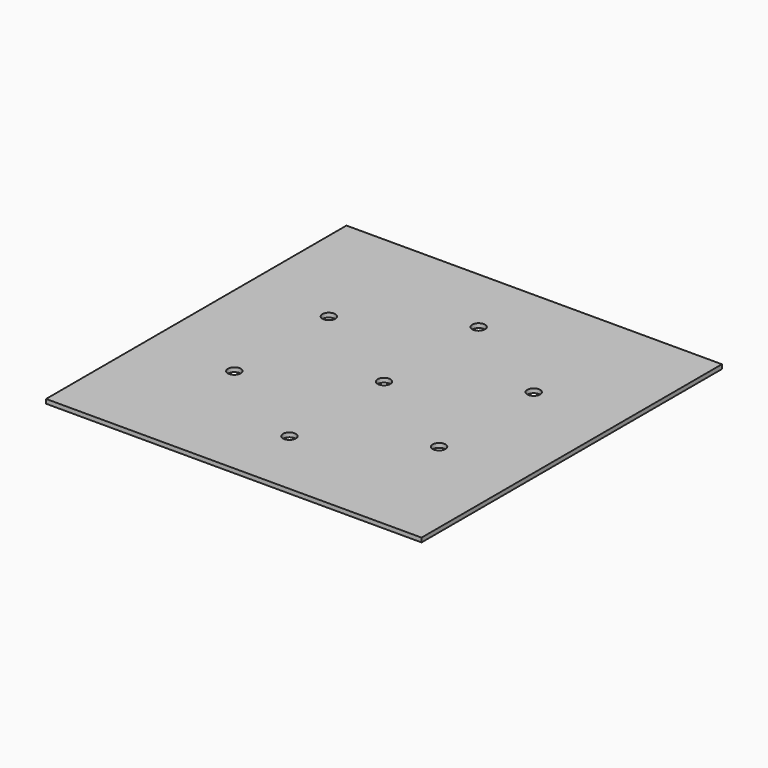
from build123d import *

# Parameters (mm, degrees)
F0_W     = 279.4
F0_H     = 279.4
F1_DEPTH = 3.175
F3_D     = 9.525


# Not quite as in the source:
# - a length typed as a fraction of an inch, garbled in the dataset ("3 / 203.2 mm" for 3/8 in), is restored


with BuildPart() as f1:
    # F0 (on Top) → F1 (new body)
    with BuildSketch(Plane.XY):
        Rectangle(F0_W, F0_H)
    extrude(amount=F1_DEPTH)

    # F3 (through all)
    with Locations(Plane.XY.offset(3.175)):
        with Locations((0, 87.9881810245), (76.2, 43.9940905122), (76.2, -43.9940905122), (0, -87.9881810245), (-76.2, -43.9940905122), (-76.2, 43.9940905122), (0, 0)):
            Hole(F3_D / 2)


solid = f1.part
